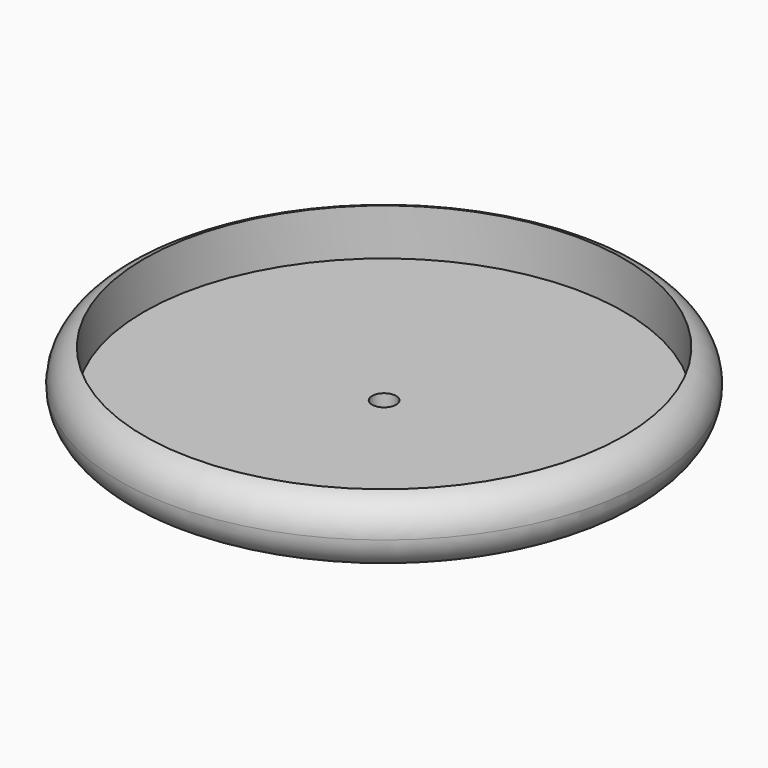
from build123d import *

# Parameters (mm, degrees)
F0_R           = 110
F1_DEPTH       = 28
F2_R           = 13.99999
F3_R           = 100
F4_DEPTH       = 20
F6_D           = 10
F6_CSINK_D     = 12.5
F6_CSINK_ANGLE = 90


# Not quite as in the source:
# - a fillet or chamfer is up to 0.001 mm smaller than in the source, because OpenCascade refuses the exact size


with BuildPart() as f1:
    # F0 (on Top) → F1 (new body)
    with BuildSketch(Plane.XY):
        Circle(F0_R)
    extrude(amount=F1_DEPTH)

    # F2 (radius 14 in the source; OpenCascade refuses exactly that, so slightly less here)
    f2_edges = [f1.edges().sort_by_distance(p)[0] for p in [
        (-110, 0, 28),
        (-110, 0, 0),
    ]]
    fillet(f2_edges, radius=F2_R)

    # F3 (on face) → F4 (cut)
    with BuildSketch(Plane.XY.offset(28)):
        Circle(F3_R)
    extrude(amount=-F4_DEPTH, mode=Mode.SUBTRACT)

    # F6 (through all)
    with Locations(Plane(origin=(0, 0, 0), x_dir=(1, 0, 0), z_dir=(0, 0, -1))):
        with Locations((0, 0)):
            CounterSinkHole(F6_D / 2, F6_CSINK_D / 2, counter_sink_angle=F6_CSINK_ANGLE)


solid = f1.part
